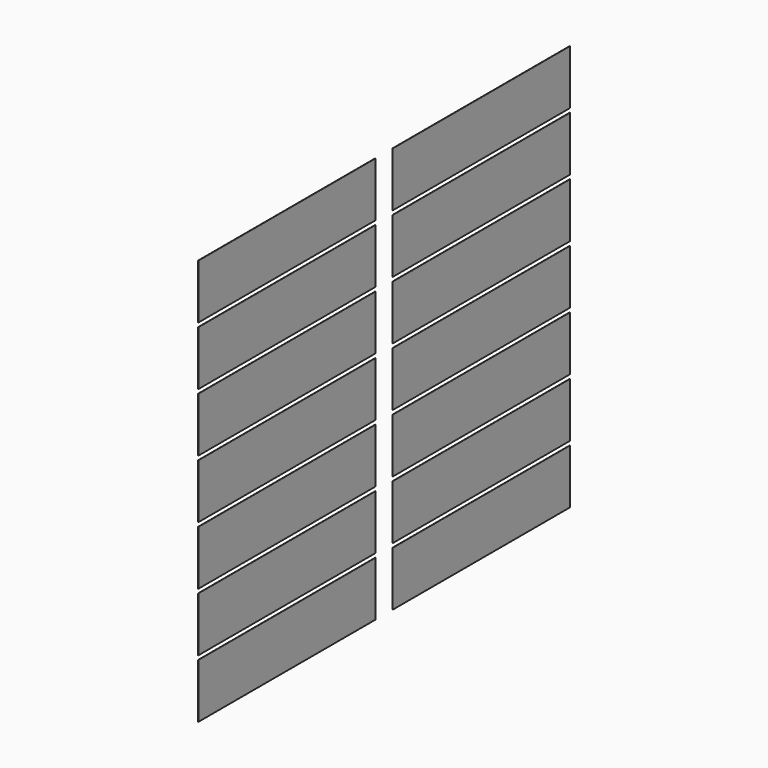
from build123d import *

# Parameters (mm, degrees)
F1_DEPTH = 0.012


# Not quite as in the source:
# - a feature names something its author has since deleted; it is built from what else it names


with BuildPart() as f1:
    # F0 (on Right) → F1 (new body)
    with BuildSketch(Plane.YZ):
        Polygon((14.3471, -0.6521), (0.6521, -0.6521), (0.6521, -2.2088), (0.6521, -2.4638), (0.6521, -4.0238), (14.3471, -4.0238), (14.3471, -2.4638), (14.3471, -2.2088), align=None)
    extrude(amount=F1_DEPTH)


with BuildPart() as f1b:
    # F0 (on Right) → F1, piece 2 (new body)
    with BuildSketch(Plane.YZ):
        Polygon((14.3471, -4.2738), (0.6521, -4.2738), (0.6521, -5.8338), (0.6521, -6.0838), (0.6521, -7.6438), (14.3471, -7.6438), (14.3471, -6.0838), (14.3471, -5.8338), align=None)
    extrude(amount=F1_DEPTH)


with BuildPart() as f1c:
    # F0 (on Right) → F1, piece 3 (new body)
    with BuildSketch(Plane.YZ):
        Polygon((14.3471, -11.5138), (0.6521, -11.5138), (0.6521, -13.0738), (0.6521, -13.3238), (0.6521, -14.8838), (14.3471, -14.8838), (14.3471, -13.3238), (14.3471, -13.0738), align=None)
    extrude(amount=F1_DEPTH)


with BuildPart() as f1d:
    # F0 (on Right) → F1, piece 4 (new body)
    with BuildSketch(Plane.YZ):
        Polygon((14.3471, -7.8938), (0.6521, -7.8938), (0.6521, -9.4538), (0.6521, -9.7038), (0.6521, -11.2638), (14.3471, -11.2638), (14.3471, -9.7038), (14.3471, -9.4538), align=None)
    extrude(amount=F1_DEPTH)


with BuildPart() as f1e:
    # F0 (on Right) → F1, piece 5 (new body)
    with BuildSketch(Plane.YZ):
        Polygon((14.3471, -15.1338), (0.6521, -15.1338), (0.6521, -16.6938), (0.6521, -18.5038), (14.3471, -18.5038), (14.3471, -16.9438), (14.3471, -16.6938), align=None)
    extrude(amount=F1_DEPTH)


with BuildPart() as f1f:
    # F0 (on Right) → F1, piece 6 (new body)
    with BuildSketch(Plane.YZ):
        Polygon((14.3471, -18.7538), (0.6521, -18.7538), (0.6521, -20.3138), (0.6521, -20.5638), (0.6521, -22.1238), (14.3471, -22.1238), (14.3471, -20.5638), (14.3471, -20.3138), align=None)
    extrude(amount=F1_DEPTH)


with BuildPart() as f1g:
    # F0 (on Right) → F1, piece 7 (new body)
    with BuildSketch(Plane.YZ):
        Polygon((14.3471, -22.3738), (0.6521, -22.3738), (0.6521, -23.9338), (0.6521, -24.1838), (0.6521, -25.7438), (14.3471, -25.7438), (14.3471, -24.1838), (14.3471, -23.9338), align=None)
    extrude(amount=F1_DEPTH)


with BuildPart() as f1h:
    # F0 (on Right) → F1, piece 8 (new body)
    with BuildSketch(Plane.YZ):
        Polygon((29.3479, -22.3738), (15.6529, -22.3738), (15.6529, -23.9338), (15.6529, -24.1838), (15.6529, -25.7438), (29.3479, -25.7438), (29.3479, -24.1838), (29.3479, -23.9338), align=None)
    extrude(amount=F1_DEPTH)


with BuildPart() as f1i:
    # F0 (on Right) → F1, piece 9 (new body)
    with BuildSketch(Plane.YZ):
        Polygon((29.3479, -7.6438), (29.3479, -6.0838), (29.3479, -5.8338), (29.3479, -4.2738), (15.6529, -4.2738), (15.6529, -5.8338), (15.6529, -6.0838), (15.6529, -7.6438), align=None)
    extrude(amount=F1_DEPTH)


with BuildPart() as f1j:
    # F0 (on Right) → F1, piece 10 (new body)
    with BuildSketch(Plane.YZ):
        Polygon((29.3479, -9.4538), (29.3479, -7.8938), (15.6529, -7.8938), (15.6529, -9.4538), (15.6529, -9.7038), (15.6529, -11.2638), (29.3479, -11.2638), (29.3479, -9.7038), align=None)
    extrude(amount=F1_DEPTH)


with BuildPart() as f1k:
    # F0 (on Right) → F1, piece 11 (new body)
    with BuildSketch(Plane.YZ):
        Polygon((29.3479, -13.0738), (29.3479, -11.5138), (15.6529, -11.5138), (15.6529, -13.0738), (15.6529, -13.3238), (15.6529, -14.8838), (29.3479, -14.8838), (29.3479, -13.3238), align=None)
    extrude(amount=F1_DEPTH)


with BuildPart() as f1l:
    # F0 (on Right) → F1, piece 12 (new body)
    with BuildSketch(Plane.YZ):
        Polygon((29.3479, -22.1238), (29.3479, -20.5638), (29.3479, -20.3138), (29.3479, -18.7538), (15.6529, -18.7538), (15.6529, -20.3138), (15.6529, -20.5638), (15.6529, -22.1238), align=None)
    extrude(amount=F1_DEPTH)


with BuildPart() as f1m:
    # F0 (on Right) → F1, piece 13 (new body)
    with BuildSketch(Plane.YZ):
        Polygon((15.6529, -15.1338), (15.6529, -16.6938), (15.6529, -16.9438), (15.6529, -18.5038), (29.3479, -18.5038), (29.3479, -16.6938), (29.3479, -15.1338), align=None)
    extrude(amount=F1_DEPTH)


with BuildPart() as f1n:
    # F0 (on Right) → F1, piece 14 (new body)
    with BuildSketch(Plane.YZ):
        Polygon((29.3479, -2.2088), (29.3479, -0.6521), (15.6529, -0.6521), (15.6529, -2.2088), (15.6529, -2.4638), (15.6529, -4.0238), (29.3479, -4.0238), (29.3479, -2.4638), align=None)
    extrude(amount=F1_DEPTH)


solid = Compound([f1.part, f1b.part, f1c.part, f1d.part, f1e.part, f1f.part, f1g.part, f1h.part, f1i.part, f1j.part, f1k.part, f1l.part, f1m.part, f1n.part])
